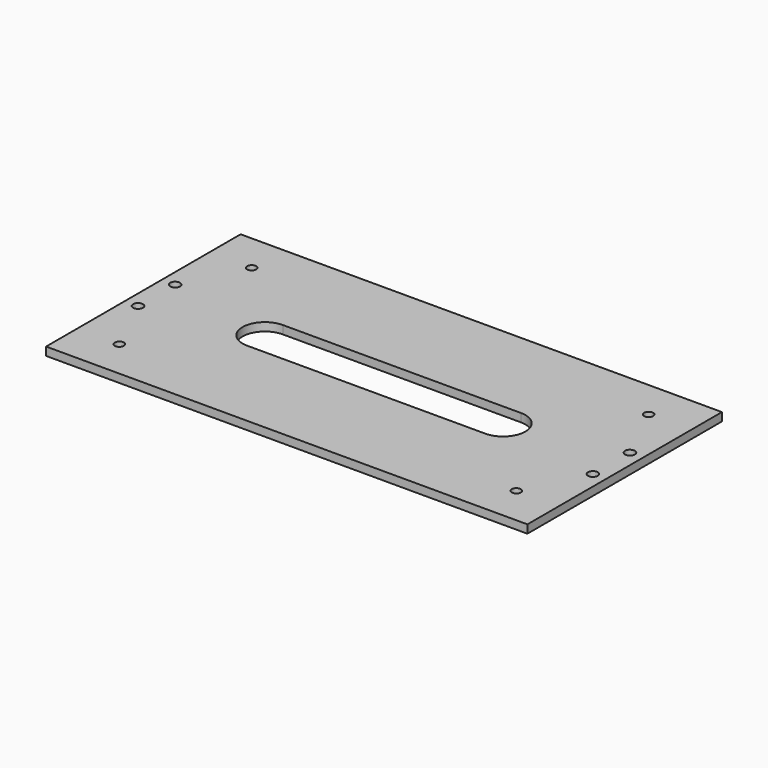
from build123d import *

# Parameters (mm, degrees)
F2_W     = 291
F2_H     = 147
F3_DEPTH = 5
F5_D     = 5.5
F6_R     = 3
F7_DEPTH = 5.001


# Not quite as in the source:
# - a pattern or mirror of a feature is missing from the dataset's text; its kind, count and spacing are read off the source's solid


with BuildPart() as f3:
    # F2 (on Top) → F3 (new body)
    with BuildSketch(Plane.XY):
        Rectangle(F2_W, F2_H)
        with BuildLine():
            ThreePointArc((-72, -13.5), (-85.5, 0), (-72, 13.5))
            Line((-72, 13.5), (72, 13.5))
            ThreePointArc((72, 13.5), (85.5, 0), (72, -13.5))
            Line((72, -13.5), (-72, -13.5))
        make_face(mode=Mode.SUBTRACT)
    extrude(amount=-F3_DEPTH)

    # F5 (through all)
    with Locations(Plane.XY):
        with Locations((-120, -50)):
            f5 = Hole(F5_D / 2)

    # F5_copies: F5 across plane
    add(f5.mirror(Plane(origin=(0, 0, 0), x_dir=(0, 0, 1), z_dir=(1, 0, 0))), mode=Mode.SUBTRACT)

    # F5_copies1: F5 across plane
    add(f5.mirror(Plane.ZX), mode=Mode.SUBTRACT)

    # F5_copies2: F5 across plane
    add(f5.mirror(Plane(origin=(0, 0, 0), x_dir=(-0.3846153846, 0.9230769231, 0), z_dir=(0.9230769231, 0.3846153846, 0))), mode=Mode.SUBTRACT)

    # F6 (on Top) → F7 (cut, through all)
    with BuildSketch(Plane.XY):
        with Locations((-137.5, -14)):
            Circle(F6_R)
    f7 = extrude(amount=-F7_DEPTH, mode=Mode.SUBTRACT)

    # F7_copies: F7 across plane
    add(f7.mirror(Plane(origin=(0, 0, 0), x_dir=(0, 0, 1), z_dir=(1, 0, 0))), mode=Mode.SUBTRACT)

    # F7_copies1: F7 across plane
    add(f7.mirror(Plane.ZX), mode=Mode.SUBTRACT)

    # F7_copies2: F7 across plane
    add(f7.mirror(Plane(origin=(0, 0, 0), x_dir=(-0.1012944786, 0.9948564864, 0), z_dir=(0.9948564864, 0.1012944786, 0))), mode=Mode.SUBTRACT)


solid = f3.part
